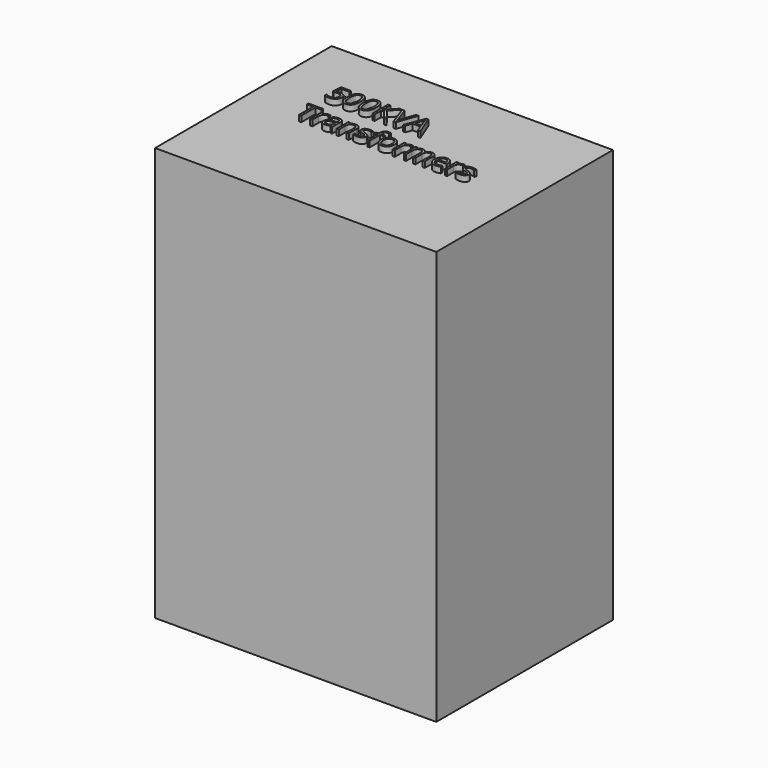
from build123d import *

# Parameters (mm, degrees)
F0_W         = 1225.804
F0_H         = 962.406
F1_DEPTH     = 1803.4
F2_TEXT_SIZE = 119.9026381137
F3_DEPTH     = 25.4


# Not quite as in the source:
# - Text() gives the source's letters only with a copy of the font that has no kerning and outlines rounded to 1/6400 em; it was checked with that copy


with BuildPart() as f1:
    # F0 (on Top) → F1 (new body)
    with BuildSketch(Plane.XY):
        Rectangle(F0_W, F0_H)
    extrude(amount=F1_DEPTH)

    # F2 (on face) → F3 (join)
    with BuildSketch(Plane.XY.offset(1803.4)):
        with Locations((-381, 140.8731005581)):
            Text('500KVA', F2_TEXT_SIZE, font='Open Sans', text_align=(TextAlign.LEFT, TextAlign.BOTTOM))
        with Locations((-381, -22.1944872766)):
            Text('Transformers', F2_TEXT_SIZE, font='Open Sans', text_align=(TextAlign.LEFT, TextAlign.BOTTOM))
    extrude(amount=F3_DEPTH)


solid = f1.part
